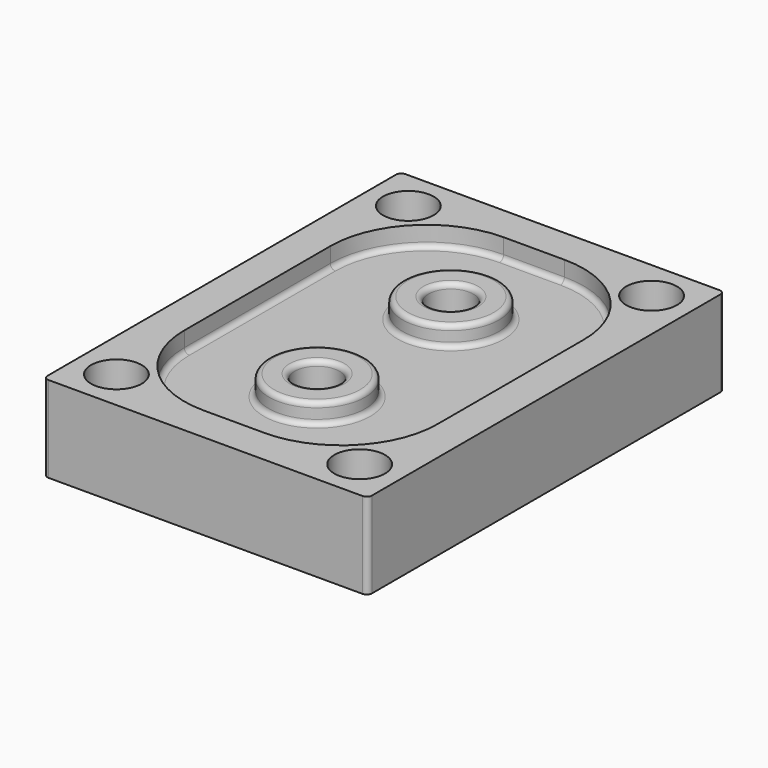
from build123d import *

# Parameters (mm, degrees)
F0_W     = 64
F0_H     = 88
F1_DEPTH = 17
F3_D     = 10
F4_W     = 28
F4_H     = 60
F5_DEPTH = 4
F7_D     = 8.8
F8_R     = 9.5
F9_DEPTH = 4
F10_R    = 1


# Not quite as in the source:
# - two fillets or chamfers of one size are made in one step


with BuildPart() as f1:
    # F0 (on Top) → F1 (new body)
    with BuildSketch(Plane.XY):
        Rectangle(F0_W, F0_H)
    extrude(amount=F1_DEPTH)

    # F3 (through all)
    with Locations(Plane(origin=(0, 0, 0), x_dir=(1, 0, 0), z_dir=(0, 0, -1))):
        with Locations((-24, -36), (24, -36), (24, 36), (-24, 36)):
            Hole(F3_D / 2)

    # F4 (on Top) → F5 (cut)
    with BuildSketch(Plane.XY):
        Rectangle(F4_W, F4_H)
    extrude(amount=F5_DEPTH, mode=Mode.SUBTRACT)

    # F7 (through all)
    with Locations(Plane(origin=(0, 0, 0), x_dir=(1, 0, 0), z_dir=(0, 0, -1))):
        with Locations((0, 16.5), (0, -16.5)):
            Hole(F7_D / 2)

    # F8 (on face) → F9 (cut)
    with BuildSketch(Plane.XY.offset(17)):
        with BuildLine():
            ThreePointArc((-6, 37), (-19.4350288425, 31.4350288425), (-25, 18))
            Line((-25, 18), (-25, 0))
            Line((-25, 0), (-25, -18))
            ThreePointArc((-25, -18), (-19.4350288425, -31.4350288425), (-6, -37))
            Line((-6, -37), (0, -37))
            Line((0, -37), (6, -37))
            ThreePointArc((6, -37), (19.4350288425, -31.4350288425), (25, -18))
            Line((25, -18), (25, 0))
            Line((25, 0), (25, 18))
            ThreePointArc((25, 18), (19.4350288425, 31.4350288425), (6, 37))
            Line((6, 37), (0, 37))
            Line((0, 37), (-6, 37))
        make_face()
        with Locations((0, -16.5)):
            Circle(F8_R, mode=Mode.SUBTRACT)
        with Locations((0, 16.5)):
            Circle(F8_R, mode=Mode.SUBTRACT)
    extrude(amount=-F9_DEPTH, mode=Mode.SUBTRACT)

    # F10
    f10_edges = [f1.edges().sort_by_distance(p)[0] for p in [
        (19.435029, 31.435029, 13),
        (0, 37, 13),
        (-19.435029, 31.435029, 13),
        (-25, 0, 13),
        (-19.435029, -31.435029, 13),
        (0, -37, 13),
        (19.435029, -31.435029, 13),
        (25, 0, 13),
        (-9.5, -16.5, 13),
        (-9.5, 16.5, 13),
        (-9.5, -16.5, 17),
        (-4.4, -16.5, 17),
        (-9.5, 16.5, 17),
        (-4.4, 16.5, 17),
        (32, 44, 8.5),
        (-32, 44, 8.5),
        (32, -44, 8.5),
        (-32, -44, 8.5),
    ]]
    fillet(f10_edges, radius=F10_R)


solid = f1.part
